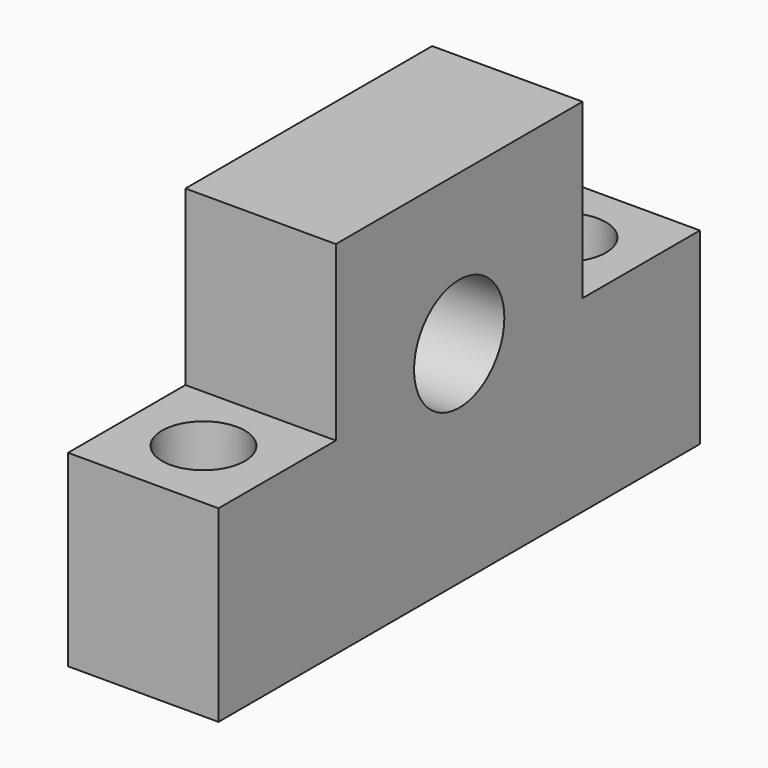
from build123d import *

# Parameters (mm, degrees)
F0_W     = 80
F0_H     = 48
F1_DEPTH = 20
F2_R     = 7.5
F3_DEPTH = 20.001
F4_W     = 19.5
F4_H     = 23
F5_DEPTH = 20.001
F6_R     = 5.5
F6_R_2   = 4
F7_DEPTH = 6
F8_DEPTH = 25.001


with BuildPart() as f1:
    # F0 (on Right) → F1 (new body)
    with BuildSketch(Plane.YZ):
        Rectangle(F0_W, F0_H)
    extrude(amount=F1_DEPTH)

    # F2 (on face) → F3 (cut, through all)
    with BuildSketch(Plane.YZ.offset(20)):
        with Locations((0, 4)):
            Circle(F2_R)
    extrude(amount=-F3_DEPTH, mode=Mode.SUBTRACT)

    # F4 (on face) → F5 (cut, through all)
    with BuildSketch(Plane.YZ.offset(20)):
        with Locations((-30.25, 12.5)):
            Rectangle(F4_W, F4_H)
        with Locations((30.25, 12.5)):
            Rectangle(F4_W, F4_H)
    extrude(amount=-F5_DEPTH, mode=Mode.SUBTRACT)

    # F6 (on face) → F7 (cut)
    with BuildSketch(Plane.XY.offset(1)):
        with Locations((10, 30)):
            Circle(F6_R)
        with Locations((10, 30)):
            Circle(F6_R_2, mode=Mode.SUBTRACT)
        with Locations((10, -30)):
            Circle(F6_R)
        with Locations((10, -30)):
            Circle(F6_R_2, mode=Mode.SUBTRACT)
    extrude(amount=-F7_DEPTH, mode=Mode.SUBTRACT)

    # F8 (cut, through all): faces of the model
    f8_faces = [f1.faces().sort_by_distance(p)[0] for p in [
        (10, 30, 1),
        (10, -30, 1),
    ]]
    extrude(f8_faces, amount=-F8_DEPTH, mode=Mode.SUBTRACT)


solid = f1.part
